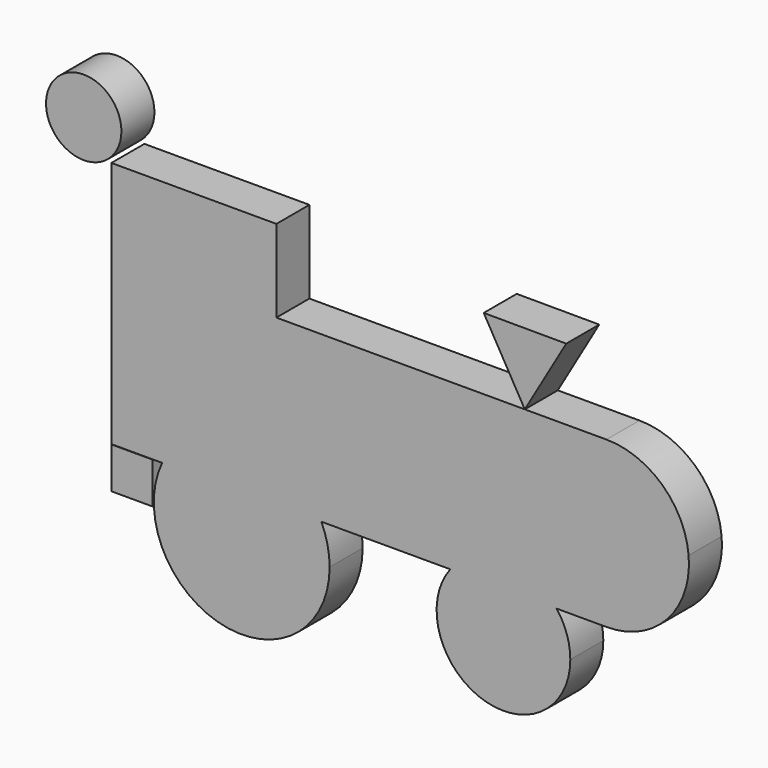
from build123d import *

# Parameters (mm, degrees)
F1_W     = 50.8
F1_H     = 25.4
F2_DEPTH = 12.7
F1_W_2   = 12.7
F1_H_2   = 12.7
F0_R     = 11.6061953028


with BuildPart() as f2:
    # F1 (on Front) → F2 (new body)
    with BuildSketch(Plane.XZ):
        with Locations((-26.0346938372, 35.8717816622)):
            Rectangle(F1_W, F1_H)
        with BuildLine():
            Line((-0.6346938372, 23.1717816622), (-51.4346938372, 23.1717816622))
            Line((-51.4346938372, 23.1717816622), (-51.4346938372, -27.6282183378))
            Line((-51.4346938372, -27.6282183378), (-35.8106568949, -27.6282183378))
            ThreePointArc((-35.8106568949, -27.6282183378), (-11.3088339567, -12.0524939981), (13.1929889814, -27.6282183378))
            Line((13.1929889814, -27.6282183378), (52.8828968769, -27.6282183378))
            ThreePointArc((52.8828968769, -27.6282183378), (69.2636594176, -19.5055942382), (85.6444219583, -27.6282183378))
            Line((85.6444219583, -27.6282183378), (100.9653061628, -27.6282183378))
            Line((100.9653061628, -27.6282183378), (100.9653061628, 23.1717816622))
            Line((100.9653061628, 23.1717816622), (75.827864427, 23.1717816622))
            Line((75.827864427, 23.1717816622), (-0.6346938372, 23.1717816622))
        make_face()
        with BuildLine():
            ThreePointArc((13.1929889814, -27.6282183378), (-11.3088339567, -12.0524939981), (-35.8106568949, -27.6282183378))
            Line((-35.8106568949, -27.6282183378), (-11.3088339567, -27.6282183378))
            Line((-11.3088339567, -27.6282183378), (13.1929889814, -27.6282183378))
        make_face()
        with BuildLine():
            Line((-11.3088339567, -27.6282183378), (-35.8106568949, -27.6282183378))
            ThreePointArc((-35.8106568949, -27.6282183378), (-17.1914081512, -65.5243298477), (15.7506625268, -39.1119904816))
            ThreePointArc((15.7506625268, -39.1119904816), (15.1035054093, -33.2294162871), (13.1929889814, -27.6282183378))
            Line((13.1929889814, -27.6282183378), (-11.3088339567, -27.6282183378))
        make_face()
        with BuildLine():
            ThreePointArc((126.2673820271, 0), (118.1199448098, 16.5035293887), (100.9653061628, 23.1717816622))
            Line((100.9653061628, 23.1717816622), (100.9653061628, -27.6282183378))
            ThreePointArc((100.9653061628, -27.6282183378), (119.6970538894, -19.3828569848), (126.2673820271, 0))
        make_face()
        with BuildLine():
            ThreePointArc((85.6444219583, -27.6282183378), (69.2636594176, -19.5055942382), (52.8828968769, -27.6282183378))
            Line((52.8828968769, -27.6282183378), (85.6444219583, -27.6282183378))
        make_face()
        with BuildLine():
            Line((85.6444219583, -27.6282183378), (52.8828968769, -27.6282183378))
            ThreePointArc((52.8828968769, -27.6282183378), (62.6914232933, -59.5853239072), (89.8423787807, -40.0843136013))
            ThreePointArc((89.8423787807, -40.0843136013), (88.7646697236, -33.512077477), (85.6444219583, -27.6282183378))
        make_face()
    extrude(amount=F2_DEPTH)


with BuildPart() as f2b:
    # F1 (on Front) → F2, piece 2 (new body)
    with BuildSketch(Plane.XZ):
        Polygon((63.1885279137, 45.2037396438), (75.827864427, 23.1717816622), (88.5884314775, 45.1337471604), align=None)
    extrude(amount=F2_DEPTH)


with BuildPart() as f2c:
    # F1 (on Front) → F2, piece 3 (new body)
    with BuildSketch(Plane.XZ):
        with Locations((-45.11574229, -34.0687217355)):
            Rectangle(F1_W_2, F1_H_2)
    extrude(amount=F2_DEPTH)


with BuildPart() as f2d:
    # F0 (on Front) → F2, piece 4 (new body)
    with BuildSketch(Plane.XZ):
        with Locations((-59.9503405392, 58.1526570022)):
            Circle(F0_R)
    extrude(amount=F2_DEPTH)


solid = Compound([f2.part, f2b.part, f2c.part, f2d.part])
